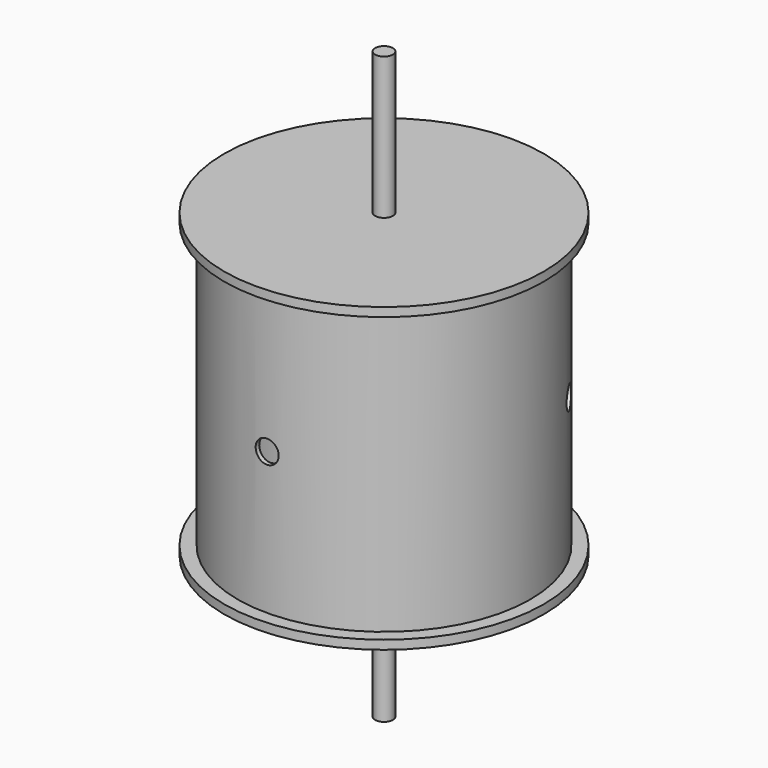
from build123d import *

# Parameters (mm, degrees)
F0_R            = 82.5
F0_R_2          = 80
F1_DEPTH        = 80
F0_R_3          = 90
F3_DEPTH        = 5
F7_D            = 13
F7_DEPTH        = 3.175
F7_TIP          = 3.9055940237
F7_COPIES_COUNT = 3
F8_R            = 5
F9_DEPTH        = 80
F9_DEPTH_BACK   = 250


# Not quite as in the source:
# - a pattern or mirror of a feature is missing from the dataset's text; its kind, count and spacing are read off the source's solid


with BuildPart() as f1:
    # F0 (on Top) → F1 (new body)
    with BuildSketch(Plane.XY):
        Circle(F0_R)
        Circle(F0_R_2, mode=Mode.SUBTRACT)
    extrude(amount=F1_DEPTH)

    # F4: F1, F3 across plane


with BuildPart() as f3:
    # F0 (on Top) → F3 (new body)
    with BuildSketch(Plane.XY):
        Circle(F0_R_3)
        Circle(F0_R, mode=Mode.SUBTRACT)
        Circle(F0_R)
        Circle(F0_R_2, mode=Mode.SUBTRACT)
        Circle(F0_R_2)
    extrude(amount=-F3_DEPTH)


with BuildPart() as f1_1:
    add(f1.part)
    add(f1.part.mirror(Plane.XY.offset(80)))
    add(f3.part.mirror(Plane.XY.offset(80)))

    # F7
    with Locations(Plane.XZ.offset(82.5)):
        with Locations((0, 80)):
            f7 = Hole(F7_D / 2, depth=F7_DEPTH)
            with Locations((0, 0, -(F7_DEPTH + F7_TIP / 2))):  # 118° drill point
                Cone(0, F7_D / 2, F7_TIP, mode=Mode.SUBTRACT)

    # F7_copies: F7 ×3 about axis
    f7_copies_axis = Axis((0, -8.6e-05, 0), (0, 0, 1))
    for i in range(1, F7_COPIES_COUNT):
        add(f7.rotate(f7_copies_axis, i * 360 / F7_COPIES_COUNT), mode=Mode.SUBTRACT)


with BuildPart() as f9:
    # F8 (on face) → F9 (new body, two sides)
    with BuildSketch(Plane.XY.offset(165)) as f9_sk:
        Circle(F8_R)
    extrude(amount=F9_DEPTH)
    extrude(f9_sk.sketch, amount=-F9_DEPTH_BACK)


solid = Compound([f3.part, f1_1.part, f9.part])
